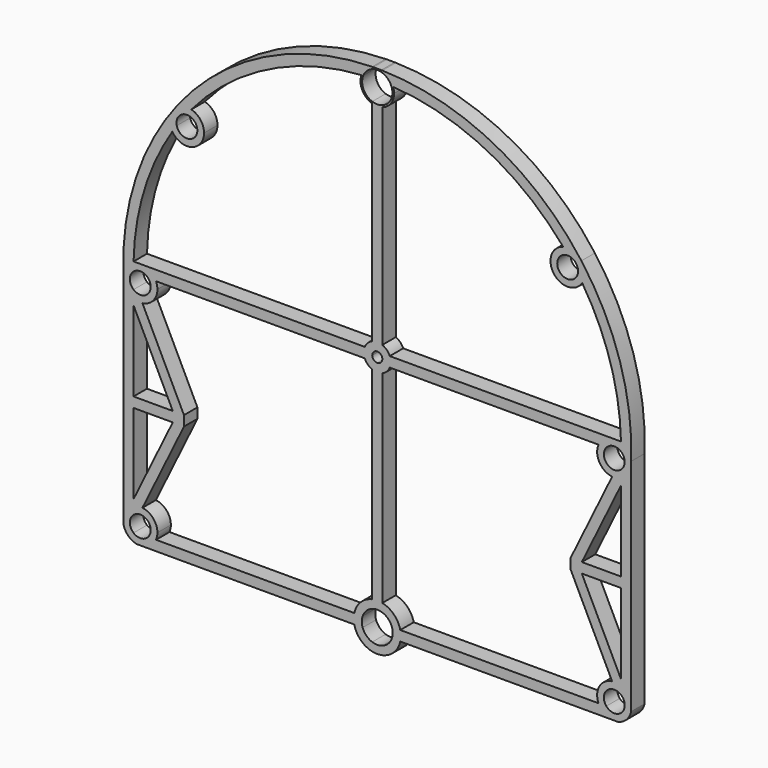
from build123d import *

# Parameters (mm, degrees)
F1_DEPTH = 5


with BuildPart() as f1:
    # F0 (on Front) → F1 (new body)
    with BuildSketch(Plane.XZ):
        with BuildLine():
            ThreePointArc((-4.749689293, 108.27741611), (-4.9150543418, 108.2746765519), (-5.080413, 108.2715751462))
            Line((-5.080413, 108.2715751462), (-5.080413, 108.1857550071))
            ThreePointArc((-5.080413, 108.1857550071), (-4.9158378094, 108.2344239279), (-4.749689293, 108.27741611))
        make_face()
        with BuildLine():
            Line((-5.080413, 108.1857550071), (-5.080413, 108.2715751462))
            ThreePointArc((-5.080413, 108.2715751462), (-38.2438547996, 99.8689539689), (-64.3052023733, 77.7053785063))
            ThreePointArc((-64.3052023733, 77.7053785063), (-61.8869598578, 79.484500638), (-58.8867953483, 79.5948878658))
            ThreePointArc((-58.8867953483, 79.5948878658), (-36.1836203834, 97.4699745631), (-8.3025955163, 105.0595285867))
            ThreePointArc((-8.3025955163, 105.0595285867), (-7.0621096732, 107.0046225393), (-5.080413, 108.1857550071))
        make_face()
        with BuildLine():
            ThreePointArc((57.1443762124, 77.7053787235), (31.0830286795, 99.8689540309), (-2.080413, 108.2715751462))
            Line((-2.080413, 108.2715751462), (-2.080413, 108.1857550071))
            ThreePointArc((-2.080413, 108.1857550071), (-0.0987163268, 107.0046225393), (1.1417695163, 105.0595285867))
            ThreePointArc((1.1417695163, 105.0595285867), (29.0227943834, 97.4699745631), (51.7259693483, 79.5948878658))
            ThreePointArc((51.7259693483, 79.5948878658), (54.7261337301, 79.4845006825), (57.1443762124, 77.7053787235))
        make_face()
        with BuildLine():
            Line((-2.080413, 108.1857550071), (-2.080413, 108.2715751462))
            ThreePointArc((-2.080413, 108.2715751462), (-2.2457716582, 108.2746765519), (-2.411136707, 108.27741611))
            ThreePointArc((-2.411136707, 108.27741611), (-2.2449881906, 108.2344239279), (-2.080413, 108.1857550071))
        make_face()
        with BuildLine():
            ThreePointArc((-4.749689293, 108.27741611), (-4.9158378094, 108.2344239279), (-5.080413, 108.1857550071))
            Line((-5.080413, 108.1857550071), (-5.080413, 107.6586996871))
            ThreePointArc((-5.080413, 107.6586996871), (-3.580413, 107.916059), (-2.080413, 107.6586996871))
            Line((-2.080413, 107.6586996871), (-2.080413, 108.1857550071))
            ThreePointArc((-2.080413, 108.1857550071), (-2.2449881906, 108.2344239279), (-2.411136707, 108.27741611))
            ThreePointArc((-2.411136707, 108.27741611), (-3.580413, 108.2864612892), (-4.749689293, 108.27741611))
        make_face()
        with BuildLine():
            Line((-5.080413, 107.6586996871), (-5.080413, 108.1857550071))
            ThreePointArc((-5.080413, 108.1857550071), (-7.0621096732, 107.0046225393), (-8.3025955163, 105.0595285867))
            ThreePointArc((-8.3025955163, 105.0595285867), (-8.0294463502, 105.0768379627), (-7.7562337923, 105.0931161579))
            ThreePointArc((-7.7562337923, 105.0931161579), (-6.6947813353, 106.6642446277), (-5.080413, 107.6586996871))
        make_face()
        with BuildLine():
            ThreePointArc((-64.5360118766, 71.9716104938), (-65.303536067, 74.8740362921), (-64.3052023733, 77.7053785063))
            ThreePointArc((-64.3052023733, 77.7053785063), (-75.7601843739, 55.1236885798), (-79.1139826123, 30.0258526184))
            ThreePointArc((-79.1139826123, 30.0258526184), (-79.0980460216, 30.1182639107), (-79.080413, 30.2103665621))
            Line((-79.080413, 30.2103665621), (-79.080413, 34.205379))
            Line((-79.080413, 34.205379), (-76.080413, 34.205379))
            Line((-76.080413, 34.205379), (-76.07297793, 34.205379))
            ThreePointArc((-76.07297793, 34.205379), (-72.9250246591, 53.8890237285), (-64.5360118766, 71.9716104938))
        make_face()
        with BuildLine():
            ThreePointArc((-58.8867953483, 79.5948878658), (-61.8869598578, 79.484500638), (-64.3052023733, 77.7053785063))
            ThreePointArc((-64.3052023733, 77.7053785063), (-65.303536067, 74.8740362921), (-64.5360118766, 71.9716104938))
            ThreePointArc((-64.5360118766, 71.9716104938), (-63.8865961541, 72.9618846049), (-63.2210941441, 73.9414205512))
            ThreePointArc((-63.2210941441, 73.9414205512), (-62.6983240118, 76.514604837), (-60.3886625308, 77.7636163754))
            ThreePointArc((-60.3886625308, 77.7636163754), (-59.6452064016, 78.6853845564), (-58.8867953483, 79.5948878658))
        make_face()
        with BuildLine():
            ThreePointArc((1.1417695163, 105.0595285867), (-0.0987163268, 107.0046225393), (-2.080413, 108.1857550071))
            Line((-2.080413, 108.1857550071), (-2.080413, 107.6586996871))
            ThreePointArc((-2.080413, 107.6586996871), (-0.4660446647, 106.6642446277), (0.5954077923, 105.0931161579))
            ThreePointArc((0.5954077923, 105.0931161579), (0.8686203502, 105.0768379627), (1.1417695163, 105.0595285867))
        make_face()
        with BuildLine():
            ThreePointArc((71.9531566123, 30.0258526184), (68.5993583338, 55.1236887089), (57.1443762124, 77.7053787235))
            ThreePointArc((57.1443762124, 77.7053787235), (57.8897416902, 76.2677404954), (58.1468371186, 74.6689048844))
            ThreePointArc((58.1468371186, 74.6689048844), (57.9501308415, 73.2661537778), (57.3751858766, 71.9716104938))
            ThreePointArc((57.3751858766, 71.9716104938), (65.7641986591, 53.8890237285), (68.91215193, 34.205379))
            Line((68.91215193, 34.205379), (68.919587, 34.205379))
            Line((68.919587, 34.205379), (71.919587, 34.205379))
            Line((71.919587, 34.205379), (71.919587, 30.2103665621))
            ThreePointArc((71.919587, 30.2103665621), (71.9372200216, 30.1182639107), (71.9531566123, 30.0258526184))
        make_face()
        with BuildLine():
            ThreePointArc((58.1468371186, 74.6689048844), (57.8897416902, 76.2677404954), (57.1443762124, 77.7053787235))
            ThreePointArc((57.1443762124, 77.7053787235), (54.7261337301, 79.4845006825), (51.7259693483, 79.5948878658))
            ThreePointArc((51.7259693483, 79.5948878658), (52.4843804016, 78.6853845564), (53.2278365308, 77.7636163754))
            ThreePointArc((53.2278365308, 77.7636163754), (55.3019533216, 76.7959805556), (56.1468371186, 74.6689048844))
            ThreePointArc((56.1468371186, 74.6689048844), (56.1251187967, 74.3025963933), (56.0602681441, 73.9414205512))
            ThreePointArc((56.0602681441, 73.9414205512), (56.7257701541, 72.9618846049), (57.3751858766, 71.9716104938))
            ThreePointArc((57.3751858766, 71.9716104938), (57.9501308415, 73.2661537778), (58.1468371186, 74.6689048844))
        make_face()
        with BuildLine():
            ThreePointArc((-7.7562337923, 105.0931161579), (-8.0294463502, 105.0768379627), (-8.3025955163, 105.0595285867))
            ThreePointArc((-8.3025955163, 105.0595285867), (-8.0481934389, 101.1713011177), (-5.080413, 98.6463629929))
            Line((-5.080413, 98.6463629929), (-5.080413, 99.1734183129))
            ThreePointArc((-5.080413, 99.1734183129), (-7.680954557, 101.5625329173), (-7.7562337923, 105.0931161579))
        make_face()
        with BuildLine():
            ThreePointArc((-55.1076631186, 74.6689048844), (-56.161280436, 77.7732223916), (-58.8867953483, 79.5948878658))
            ThreePointArc((-58.8867953483, 79.5948878658), (-59.6452064016, 78.6853845564), (-60.3886625308, 77.7636163754))
            ThreePointArc((-60.3886625308, 77.7636163754), (-58.0805874474, 76.9240210874), (-57.1076631186, 74.6689048844))
            ThreePointArc((-57.1076631186, 74.6689048844), (-59.8413546276, 71.5906232064), (-63.2210941441, 73.9414205512))
            ThreePointArc((-63.2210941441, 73.9414205512), (-63.8865961541, 72.9618846049), (-64.5360118766, 71.9716104938))
            ThreePointArc((-64.5360118766, 71.9716104938), (-58.804912012, 69.7656111615), (-55.1076631186, 74.6689048844))
        make_face()
        with BuildLine():
            ThreePointArc((1.419587, 103.416059), (1.3496434186, 104.24945189), (1.1417695163, 105.0595285867))
            ThreePointArc((1.1417695163, 105.0595285867), (0.8686203502, 105.0768379627), (0.5954077923, 105.0931161579))
            ThreePointArc((0.5954077923, 105.0931161579), (0.8377989441, 104.2701100625), (0.919587, 103.416059))
            ThreePointArc((0.919587, 103.416059), (0.0938216142, 100.8179827886), (-2.080413, 99.1734183129))
            Line((-2.080413, 99.1734183129), (-2.080413, 98.6463629929))
            ThreePointArc((-2.080413, 98.6463629929), (0.4507158741, 100.4580191085), (1.419587, 103.416059))
        make_face()
        with BuildLine():
            ThreePointArc((53.2278365308, 77.7636163754), (52.4843804016, 78.6853845564), (51.7259693483, 79.5948878658))
            ThreePointArc((51.7259693483, 79.5948878658), (48.9492982298, 71.6324307688), (57.3751858766, 71.9716104938))
            ThreePointArc((57.3751858766, 71.9716104938), (56.7257701541, 72.9618846049), (56.0602681441, 73.9414205512))
            ThreePointArc((56.0602681441, 73.9414205512), (50.5561762255, 72.8232049318), (53.2278365308, 77.7636163754))
        make_face()
        with BuildLine():
            ThreePointArc((-2.080413, 98.6463629929), (-3.580413, 98.416059), (-5.080413, 98.6463629929))
            Line((-5.080413, 98.6463629929), (-5.080413, 36.4134782435))
            ThreePointArc((-5.080413, 36.4134782435), (-3.580413, 36.705379), (-2.080413, 36.4134782435))
            Line((-2.080413, 36.4134782435), (-2.080413, 98.6463629929))
        make_face()
        with BuildLine():
            Line((-5.080413, 99.1734183129), (-5.080413, 98.6463629929))
            ThreePointArc((-5.080413, 98.6463629929), (-3.580413, 98.416059), (-2.080413, 98.6463629929))
            Line((-2.080413, 98.6463629929), (-2.080413, 99.1734183129))
            ThreePointArc((-2.080413, 99.1734183129), (-3.580413, 98.916059), (-5.080413, 99.1734183129))
        make_face()
        with BuildLine():
            ThreePointArc((-76.080413, 33.8968606423), (-78.0361126411, 32.4244534554), (-79.080413, 30.2103665621))
            Line((-79.080413, 30.2103665621), (-79.080413, 29.205379))
            Line((-79.080413, 29.205379), (-79.080413, 28.2003914379))
            ThreePointArc((-79.080413, 28.2003914379), (-78.0361126411, 25.9863045446), (-76.080413, 24.5138973577))
            Line((-76.080413, 24.5138973577), (-76.080413, 26.8368351435))
            ThreePointArc((-76.080413, 26.8368351435), (-77.180413, 29.205379), (-76.080413, 31.5739228565))
            Line((-76.080413, 31.5739228565), (-76.080413, 33.787954695))
            Line((-76.080413, 33.787954695), (-76.080413, 33.8968606423))
        make_face()
        with BuildLine():
            Line((-79.080413, 34.205379), (-79.080413, 30.2103665621))
            ThreePointArc((-79.080413, 30.2103665621), (-78.0361126411, 32.4244534554), (-76.080413, 33.8968606423))
            Line((-76.080413, 33.8968606423), (-76.080413, 34.205379))
            Line((-76.080413, 34.205379), (-79.080413, 34.205379))
        make_face()
        with BuildLine():
            ThreePointArc((-76.080413, 24.5138973577), (-78.0361126411, 25.9863045446), (-79.080413, 28.2003914379))
            Line((-79.080413, 28.2003914379), (-79.080413, -33.5006334379))
            ThreePointArc((-79.080413, -33.5006334379), (-78.0361126411, -31.2865465446), (-76.080413, -29.8141393577))
            Line((-76.080413, -29.8141393577), (-76.080413, -28.0267348672))
            Line((-76.080413, -28.0267348672), (-76.080413, -4.14996))
            Line((-76.080413, -4.14996), (-76.080413, -1.14996))
            Line((-76.080413, -1.14996), (-76.080413, 22.7268148672))
            Line((-76.080413, 22.7268148672), (-76.080413, 24.5138973577))
        make_face()
        with BuildLine():
            ThreePointArc((-76.0786929426, 33.8975935381), (-76.0759987773, 34.051489302), (-76.07297793, 34.205379))
            Line((-76.07297793, 34.205379), (-76.080413, 34.205379))
            Line((-76.080413, 34.205379), (-76.080413, 33.8968606423))
            ThreePointArc((-76.080413, 33.8968606423), (-76.0795530049, 33.897227169), (-76.0786929426, 33.8975935381))
        make_face()
        with BuildLine():
            Line((-75.0854005621, 34.205379), (-76.07297793, 34.205379))
            ThreePointArc((-76.07297793, 34.205379), (-76.0759987773, 34.051489302), (-76.0786929426, 33.8975935381))
            ThreePointArc((-76.0786929426, 33.8975935381), (-75.58991189, 34.0768688236), (-75.0854005621, 34.205379))
        make_face()
        with BuildLine():
            ThreePointArc((68.919587, 33.8968606423), (70.8752866411, 32.4244534554), (71.919587, 30.2103665621))
            Line((71.919587, 30.2103665621), (71.919587, 34.205379))
            Line((71.919587, 34.205379), (68.919587, 34.205379))
            Line((68.919587, 34.205379), (68.919587, 33.8968606423))
        make_face()
        with BuildLine():
            Line((71.919587, 29.205379), (71.919587, 30.2103665621))
            ThreePointArc((71.919587, 30.2103665621), (70.8752866411, 32.4244534554), (68.919587, 33.8968606423))
            Line((68.919587, 33.8968606423), (68.919587, 33.787954695))
            Line((68.919587, 33.787954695), (68.919587, 31.5739228565))
            ThreePointArc((68.919587, 31.5739228565), (69.7311701839, 30.5111354857), (70.019587, 29.205379))
            ThreePointArc((70.019587, 29.205379), (69.7311701839, 27.8996225143), (68.919587, 26.8368351435))
            Line((68.919587, 26.8368351435), (68.919587, 24.5138973577))
            ThreePointArc((68.919587, 24.5138973577), (70.8752866411, 25.9863045446), (71.919587, 28.2003914379))
            Line((71.919587, 28.2003914379), (71.919587, 29.205379))
        make_face()
        with BuildLine():
            ThreePointArc((-2.080413, 36.4134782435), (-3.580413, 36.705379), (-5.080413, 36.4134782435))
            Line((-5.080413, 36.4134782435), (-5.080413, 34.205379))
            Line((-5.080413, 34.205379), (-3.5804130006, 34.205379))
            Line((-3.5804130006, 34.205379), (-2.080413, 34.205379))
            Line((-2.080413, 34.205379), (-2.080413, 36.4134782435))
        make_face()
        with BuildLine():
            Line((-5.080413, 34.205379), (-5.080413, 36.4134782435))
            ThreePointArc((-5.080413, 36.4134782435), (-6.4088401247, 35.5338061247), (-7.2885122435, 34.205379))
            Line((-7.2885122435, 34.205379), (-5.080413, 34.205379))
        make_face()
        with BuildLine():
            ThreePointArc((-76.080413, -29.8141393577), (-78.0361126411, -31.2865465446), (-79.080413, -33.5006334379))
            Line((-79.080413, -33.5006334379), (-79.080413, -35.5106085621))
            ThreePointArc((-79.080413, -35.5106085621), (-78.0361126411, -37.7246954554), (-76.080413, -39.1971026423))
            Line((-76.080413, -39.1971026423), (-76.080413, -36.8741648565))
            ThreePointArc((-76.080413, -36.8741648565), (-77.180413, -34.505621), (-76.080413, -32.1370771435))
            Line((-76.080413, -32.1370771435), (-76.080413, -29.8141393577))
        make_face()
        with BuildLine():
            ThreePointArc((-73.4350428893, 24.1463773771), (-74.7822130201, 24.1538963729), (-76.080413, 24.5138973577))
            Line((-76.080413, 24.5138973577), (-76.080413, 22.7268148672))
            Line((-76.080413, 22.7268148672), (-64.4190917567, -1.14996))
            Line((-64.4190917567, -1.14996), (-61.080413, -1.14996))
            Line((-61.080413, -1.14996), (-73.4350428893, 24.1463773771))
        make_face()
        with BuildLine():
            Line((-76.080413, 26.8368351435), (-76.080413, 24.5138973577))
            ThreePointArc((-76.080413, 24.5138973577), (-74.7822130201, 24.1538963729), (-73.4350428893, 24.1463773771))
            ThreePointArc((-73.4350428893, 24.1463773771), (-70.2527905288, 25.8350220133), (-68.980413, 29.205379))
            ThreePointArc((-68.980413, 29.205379), (-69.0835861881, 30.2260267415), (-69.3889313577, 31.205379))
            Line((-69.3889313577, 31.205379), (-71.7118691435, 31.205379))
            ThreePointArc((-71.7118691435, 31.205379), (-71.1690141992, 30.2701592696), (-70.980413, 29.205379))
            ThreePointArc((-70.980413, 29.205379), (-72.7746565143, 26.3937958161), (-76.080413, 26.8368351435))
        make_face()
        with BuildLine():
            Line((-73.0754254379, 34.205379), (-75.0854005621, 34.205379))
            ThreePointArc((-75.0854005621, 34.205379), (-75.58991189, 34.0768688236), (-76.0786929426, 33.8975935381))
            ThreePointArc((-76.0786929426, 33.8975935381), (-76.0795736968, 33.8427744417), (-76.080413, 33.787954695))
            Line((-76.080413, 33.787954695), (-76.080413, 31.5739228565))
            ThreePointArc((-76.080413, 31.5739228565), (-73.8198131399, 32.2944059848), (-71.7118691435, 31.205379))
            Line((-71.7118691435, 31.205379), (-69.3889313577, 31.205379))
            ThreePointArc((-69.3889313577, 31.205379), (-70.8613385446, 33.1610786411), (-73.0754254379, 34.205379))
        make_face()
        with BuildLine():
            Line((71.919587, -33.5006334379), (71.919587, 28.2003914379))
            ThreePointArc((71.919587, 28.2003914379), (70.8752866411, 25.9863045446), (68.919587, 24.5138973577))
            Line((68.919587, 24.5138973577), (68.919587, 22.7268148672))
            Line((68.919587, 22.7268148672), (68.919587, -1.14996))
            Line((68.919587, -1.14996), (68.919587, -4.14996))
            Line((68.919587, -4.14996), (68.919587, -28.0267348672))
            Line((68.919587, -28.0267348672), (68.919587, -29.8141393577))
            ThreePointArc((68.919587, -29.8141393577), (70.8752866411, -31.2865465446), (71.919587, -33.5006334379))
        make_face()
        with BuildLine():
            ThreePointArc((68.9178669426, 33.8975935381), (68.9187270049, 33.897227169), (68.919587, 33.8968606423))
            Line((68.919587, 33.8968606423), (68.919587, 34.205379))
            Line((68.919587, 34.205379), (68.91215193, 34.205379))
            ThreePointArc((68.91215193, 34.205379), (68.9151727773, 34.051489302), (68.9178669426, 33.8975935381))
        make_face()
        with BuildLine():
            ThreePointArc((68.9178669426, 33.8975935381), (68.9151727773, 34.051489302), (68.91215193, 34.205379))
            Line((68.91215193, 34.205379), (67.9245745621, 34.205379))
            ThreePointArc((67.9245745621, 34.205379), (68.42908589, 34.0768688236), (68.9178669426, 33.8975935381))
        make_face()
        with BuildLine():
            Line((-3.5804130006, 34.205379), (-5.080413, 34.205379))
            Line((-5.080413, 34.205379), (-5.080413, 32.705379))
            ThreePointArc((-5.080413, 32.705379), (-4.641073172, 33.7660391716), (-3.5804130006, 34.205379))
        make_face()
        with BuildLine():
            Line((-5.080413, 32.705379), (-5.080413, 34.205379))
            Line((-5.080413, 34.205379), (-7.2885122435, 34.205379))
            ThreePointArc((-7.2885122435, 34.205379), (-7.580413, 32.705379), (-7.2885122435, 31.205379))
            Line((-7.2885122435, 31.205379), (-5.080413, 31.205379))
            Line((-5.080413, 31.205379), (-5.080413, 32.705379))
        make_face()
        with BuildLine():
            ThreePointArc((0.1276862435, 34.205379), (-0.7519858753, 35.5338061247), (-2.080413, 36.4134782435))
            Line((-2.080413, 36.4134782435), (-2.080413, 34.205379))
            Line((-2.080413, 34.205379), (0.1276862435, 34.205379))
        make_face()
        with BuildLine():
            ThreePointArc((-7.2885122435, 31.205379), (-7.580413, 32.705379), (-7.2885122435, 34.205379))
            Line((-7.2885122435, 34.205379), (-73.0754254379, 34.205379))
            ThreePointArc((-73.0754254379, 34.205379), (-70.8613385446, 33.1610786411), (-69.3889313577, 31.205379))
            Line((-69.3889313577, 31.205379), (-7.2885122435, 31.205379))
        make_face()
        with BuildLine():
            ThreePointArc((-73.4351909303, -29.4466004939), (-74.7822869304, -29.4541486418), (-76.080413, -29.8141393577))
            Line((-76.080413, -29.8141393577), (-76.080413, -32.1370771435))
            ThreePointArc((-76.080413, -32.1370771435), (-72.7746565143, -31.6940378161), (-70.980413, -34.505621))
            ThreePointArc((-70.980413, -34.505621), (-71.1689418324, -35.5702033783), (-71.711597284, -36.505299))
            Line((-71.711597284, -36.505299), (-69.3887941007, -36.505299))
            ThreePointArc((-69.3887941007, -36.505299), (-69.0835511655, -35.5260972647), (-68.980413, -34.505621))
            ThreePointArc((-68.980413, -34.505621), (-70.2528398423, -31.1352080101), (-73.4351909303, -29.4466004939))
        make_face()
        with BuildLine():
            Line((-76.080413, -28.0267348672), (-76.080413, -29.8141393577))
            ThreePointArc((-76.080413, -29.8141393577), (-74.7822869304, -29.4541486418), (-73.4351909303, -29.4466004939))
            Line((-73.4351909303, -29.4466004939), (-61.080413, -4.14996))
            Line((-61.080413, -4.14996), (-64.4190917567, -4.14996))
            Line((-64.4190917567, -4.14996), (-76.080413, -28.0267348672))
        make_face()
        with BuildLine():
            Line((71.919587, -35.5106085621), (71.919587, -33.5006334379))
            ThreePointArc((71.919587, -33.5006334379), (70.8752866411, -31.2865465446), (68.919587, -29.8141393577))
            Line((68.919587, -29.8141393577), (68.919587, -32.1370771435))
            ThreePointArc((68.919587, -32.1370771435), (69.7311701839, -33.1998645143), (70.019587, -34.505621))
            ThreePointArc((70.019587, -34.505621), (69.7311701839, -35.8113774857), (68.919587, -36.8741648565))
            Line((68.919587, -36.8741648565), (68.919587, -39.1971026423))
            ThreePointArc((68.919587, -39.1971026423), (70.8752866411, -37.7246954554), (71.919587, -35.5106085621))
        make_face()
        with BuildLine():
            ThreePointArc((66.2742168893, 24.1463773771), (67.6213870201, 24.1538963729), (68.919587, 24.5138973577))
            Line((68.919587, 24.5138973577), (68.919587, 26.8368351435))
            ThreePointArc((68.919587, 26.8368351435), (64.7275559783, 27.0133479783), (64.5510431435, 31.205379))
            Line((64.5510431435, 31.205379), (62.2281053577, 31.205379))
            ThreePointArc((62.2281053577, 31.205379), (62.4948980125, 26.6692150929), (66.2742168893, 24.1463773771))
        make_face()
        with BuildLine():
            Line((68.919587, 22.7268148672), (68.919587, 24.5138973577))
            ThreePointArc((68.919587, 24.5138973577), (67.6213870201, 24.1538963729), (66.2742168893, 24.1463773771))
            Line((66.2742168893, 24.1463773771), (53.919587, -1.14996))
            Line((53.919587, -1.14996), (57.2582657567, -1.14996))
            Line((57.2582657567, -1.14996), (68.919587, 22.7268148672))
        make_face()
        with BuildLine():
            Line((68.919587, 31.5739228565), (68.919587, 33.787954695))
            ThreePointArc((68.919587, 33.787954695), (68.9187476968, 33.8427744417), (68.9178669426, 33.8975935381))
            ThreePointArc((68.9178669426, 33.8975935381), (68.42908589, 34.0768688236), (67.9245745621, 34.205379))
            Line((67.9245745621, 34.205379), (65.9145994379, 34.205379))
            ThreePointArc((65.9145994379, 34.205379), (63.7005125446, 33.1610786411), (62.2281053577, 31.205379))
            Line((62.2281053577, 31.205379), (64.5510431435, 31.205379))
            ThreePointArc((64.5510431435, 31.205379), (66.6589871399, 32.2944059848), (68.919587, 31.5739228565))
        make_face()
        with BuildLine():
            ThreePointArc((-3.5804129925, 31.205379), (-4.6410731691, 31.6447188256), (-5.080413, 32.705379))
            Line((-5.080413, 32.705379), (-5.080413, 31.205379))
            Line((-5.080413, 31.205379), (-3.5804129925, 31.205379))
        make_face()
        with BuildLine():
            Line((-2.080413, 34.205379), (-3.5804130006, 34.205379))
            ThreePointArc((-3.5804130006, 34.205379), (-2.5197528284, 33.766039172), (-2.080413, 32.705379))
            Line((-2.080413, 32.705379), (-2.080413, 34.205379))
        make_face()
        with BuildLine():
            Line((0.1276862435, 34.205379), (-2.080413, 34.205379))
            Line((-2.080413, 34.205379), (-2.080413, 32.705379))
            Line((-2.080413, 32.705379), (-2.080413, 31.205379))
            Line((-2.080413, 31.205379), (0.1276862435, 31.205379))
            ThreePointArc((0.1276862435, 31.205379), (0.34593371, 31.9413099502), (0.419587, 32.705379))
            ThreePointArc((0.419587, 32.705379), (0.34593371, 33.4694480498), (0.1276862435, 34.205379))
        make_face()
        with BuildLine():
            Line((65.9145994379, 34.205379), (0.1276862435, 34.205379))
            ThreePointArc((0.1276862435, 34.205379), (0.34593371, 33.4694480498), (0.419587, 32.705379))
            ThreePointArc((0.419587, 32.705379), (0.34593371, 31.9413099502), (0.1276862435, 31.205379))
            Line((0.1276862435, 31.205379), (62.2281053577, 31.205379))
            ThreePointArc((62.2281053577, 31.205379), (63.7005125446, 33.1610786411), (65.9145994379, 34.205379))
        make_face()
        with BuildLine():
            Line((-5.080413, 31.205379), (-7.2885122435, 31.205379))
            ThreePointArc((-7.2885122435, 31.205379), (-6.4088401247, 29.8769518753), (-5.080413, 28.9972797565))
            Line((-5.080413, 28.9972797565), (-5.080413, 31.205379))
        make_face()
        with BuildLine():
            Line((-76.080413, -36.8741648565), (-76.080413, -39.1971026423))
            ThreePointArc((-76.080413, -39.1971026423), (-75.5915845549, -39.3765922103), (-75.0870012457, -39.505299))
            Line((-75.0870012457, -39.505299), (-73.0738247543, -39.505299))
            ThreePointArc((-73.0738247543, -39.505299), (-70.8605696549, -38.4606948088), (-69.3887941007, -36.505299))
            Line((-69.3887941007, -36.505299), (-71.711597284, -36.505299))
            ThreePointArc((-71.711597284, -36.505299), (-73.8196031783, -37.5946302646), (-76.080413, -36.8741648565))
        make_face()
        Polygon((-64.4190917567, -1.14996), (-76.080413, -1.14996), (-76.080413, -4.14996), (-64.4190917567, -4.14996), (-61.080413, -4.14996), (-61.080413, -1.14996), align=None)
        with BuildLine():
            ThreePointArc((66.2743649303, -29.4466004939), (67.6214609304, -29.4541486418), (68.919587, -29.8141393577))
            Line((68.919587, -29.8141393577), (68.919587, -28.0267348672))
            Line((68.919587, -28.0267348672), (57.2582657567, -4.14996))
            Line((57.2582657567, -4.14996), (53.919587, -4.14996))
            Line((53.919587, -4.14996), (66.2743649303, -29.4466004939))
        make_face()
        with BuildLine():
            Line((68.919587, -32.1370771435), (68.919587, -29.8141393577))
            ThreePointArc((68.919587, -29.8141393577), (67.6214609304, -29.4541486418), (66.2743649303, -29.4466004939))
            ThreePointArc((66.2743649303, -29.4466004939), (62.495022159, -31.9692405143), (62.2279681007, -36.505299))
            Line((62.2279681007, -36.505299), (64.550771284, -36.505299))
            ThreePointArc((64.550771284, -36.505299), (64.7277049765, -32.3134409903), (68.919587, -32.1370771435))
        make_face()
        with BuildLine():
            Line((-3.5804129925, 31.205379), (-5.080413, 31.205379))
            Line((-5.080413, 31.205379), (-5.080413, 28.9972797565))
            ThreePointArc((-5.080413, 28.9972797565), (-3.580413, 28.705379), (-2.080413, 28.9972797565))
            Line((-2.080413, 28.9972797565), (-2.080413, 31.205379))
            Line((-2.080413, 31.205379), (-3.5804129925, 31.205379))
        make_face()
        with BuildLine():
            ThreePointArc((-2.080413, 32.705379), (-2.5197528256, 31.6447188309), (-3.5804129925, 31.205379))
            Line((-3.5804129925, 31.205379), (-2.080413, 31.205379))
            Line((-2.080413, 31.205379), (-2.080413, 32.705379))
        make_face()
        with BuildLine():
            ThreePointArc((-2.080413, 28.9972797565), (-3.580413, 28.705379), (-5.080413, 28.9972797565))
            Line((-5.080413, 28.9972797565), (-5.080413, -31.1679018344))
            ThreePointArc((-5.080413, -31.1679018344), (-3.580413, -31.005299), (-2.080413, -31.1679018344))
            Line((-2.080413, -31.1679018344), (-2.080413, 28.9972797565))
        make_face()
        with BuildLine():
            ThreePointArc((67.9261752457, -39.505299), (68.4307585549, -39.3765922103), (68.919587, -39.1971026423))
            Line((68.919587, -39.1971026423), (68.919587, -36.8741648565))
            ThreePointArc((68.919587, -36.8741648565), (66.6587771783, -37.5946302646), (64.550771284, -36.505299))
            Line((64.550771284, -36.505299), (62.2279681007, -36.505299))
            ThreePointArc((62.2279681007, -36.505299), (63.6997436549, -38.4606948088), (65.9129987543, -39.505299))
            Line((65.9129987543, -39.505299), (67.9261752457, -39.505299))
        make_face()
        Polygon((68.919587, -4.14996), (68.919587, -1.14996), (57.2582657567, -1.14996), (53.919587, -1.14996), (53.919587, -4.14996), (57.2582657567, -4.14996), align=None)
        with BuildLine():
            Line((0.1276862435, 31.205379), (-2.080413, 31.205379))
            Line((-2.080413, 31.205379), (-2.080413, 28.9972797565))
            ThreePointArc((-2.080413, 28.9972797565), (-0.7519858753, 29.8769518753), (0.1276862435, 31.205379))
        make_face()
        with BuildLine():
            ThreePointArc((-2.080413, -31.1679018344), (-3.580413, -31.005299), (-5.080413, -31.1679018344))
            Line((-5.080413, -31.1679018344), (-5.080413, -33.656736019))
            ThreePointArc((-5.080413, -33.656736019), (-3.580413, -33.405299), (-2.080413, -33.656736019))
            Line((-2.080413, -33.656736019), (-2.080413, -31.1679018344))
        make_face()
        with BuildLine():
            Line((-5.080413, -33.656736019), (-5.080413, -31.1679018344))
            ThreePointArc((-5.080413, -31.1679018344), (-8.5301604683, -33.0555515317), (-10.4178101656, -36.505299))
            Line((-10.4178101656, -36.505299), (-7.928975981, -36.505299))
            ThreePointArc((-7.928975981, -36.505299), (-6.8331041935, -34.7526078065), (-5.080413, -33.656736019))
        make_face()
        with BuildLine():
            ThreePointArc((-69.3887941007, -36.505299), (-70.8605696549, -38.4606948088), (-73.0738247543, -39.505299))
            Line((-73.0738247543, -39.505299), (-10.4178101656, -39.505299))
            ThreePointArc((-10.4178101656, -39.505299), (-10.580413, -38.005299), (-10.4178101656, -36.505299))
            Line((-10.4178101656, -36.505299), (-69.3887941007, -36.505299))
        make_face()
        with BuildLine():
            ThreePointArc((65.9129987543, -39.505299), (63.6997436549, -38.4606948088), (62.2279681007, -36.505299))
            Line((62.2279681007, -36.505299), (3.2569841656, -36.505299))
            ThreePointArc((3.2569841656, -36.505299), (3.3788175666, -37.2509052564), (3.419587, -38.005299))
            ThreePointArc((3.419587, -38.005299), (3.3788175666, -38.7596927436), (3.2569841656, -39.505299))
            Line((3.2569841656, -39.505299), (65.9129987543, -39.505299))
        make_face()
        with BuildLine():
            ThreePointArc((3.2569841656, -36.505299), (1.3693344683, -33.0555515317), (-2.080413, -31.1679018344))
            Line((-2.080413, -31.1679018344), (-2.080413, -33.656736019))
            ThreePointArc((-2.080413, -33.656736019), (-0.3277218065, -34.7526078065), (0.768149981, -36.505299))
            Line((0.768149981, -36.505299), (3.2569841656, -36.505299))
        make_face()
        with BuildLine():
            Line((-7.928975981, -36.505299), (-10.4178101656, -36.505299))
            ThreePointArc((-10.4178101656, -36.505299), (-10.580413, -38.005299), (-10.4178101656, -39.505299))
            Line((-10.4178101656, -39.505299), (-7.928975981, -39.505299))
            ThreePointArc((-7.928975981, -39.505299), (-8.180413, -38.005299), (-7.928975981, -36.505299))
        make_face()
        with BuildLine():
            Line((-7.928975981, -39.505299), (-10.4178101656, -39.505299))
            ThreePointArc((-10.4178101656, -39.505299), (-8.5301604683, -42.9550464683), (-5.080413, -44.8426961656))
            Line((-5.080413, -44.8426961656), (-5.080413, -42.353861981))
            ThreePointArc((-5.080413, -42.353861981), (-6.8331041935, -41.2579901935), (-7.928975981, -39.505299))
        make_face()
        with BuildLine():
            ThreePointArc((3.419587, -38.005299), (3.3788175666, -37.2509052564), (3.2569841656, -36.505299))
            Line((3.2569841656, -36.505299), (0.768149981, -36.505299))
            ThreePointArc((0.768149981, -36.505299), (0.9562922865, -37.2448352312), (1.019587, -38.005299))
            ThreePointArc((1.019587, -38.005299), (0.9562922865, -38.7657627688), (0.768149981, -39.505299))
            Line((0.768149981, -39.505299), (3.2569841656, -39.505299))
            ThreePointArc((3.2569841656, -39.505299), (3.3788175666, -38.7596927436), (3.419587, -38.005299))
        make_face()
        with BuildLine():
            Line((-5.080413, -42.353861981), (-5.080413, -44.8426961656))
            ThreePointArc((-5.080413, -44.8426961656), (-3.580413, -45.005299), (-2.080413, -44.8426961656))
            Line((-2.080413, -44.8426961656), (-2.080413, -42.353861981))
            ThreePointArc((-2.080413, -42.353861981), (-3.580413, -42.605299), (-5.080413, -42.353861981))
        make_face()
        with BuildLine():
            ThreePointArc((-2.080413, -44.8426961656), (1.3693344683, -42.9550464683), (3.2569841656, -39.505299))
            Line((3.2569841656, -39.505299), (0.768149981, -39.505299))
            ThreePointArc((0.768149981, -39.505299), (-0.3277218065, -41.2579901935), (-2.080413, -42.353861981))
            Line((-2.080413, -42.353861981), (-2.080413, -44.8426961656))
        make_face()
    extrude(amount=F1_DEPTH)


solid = f1.part
